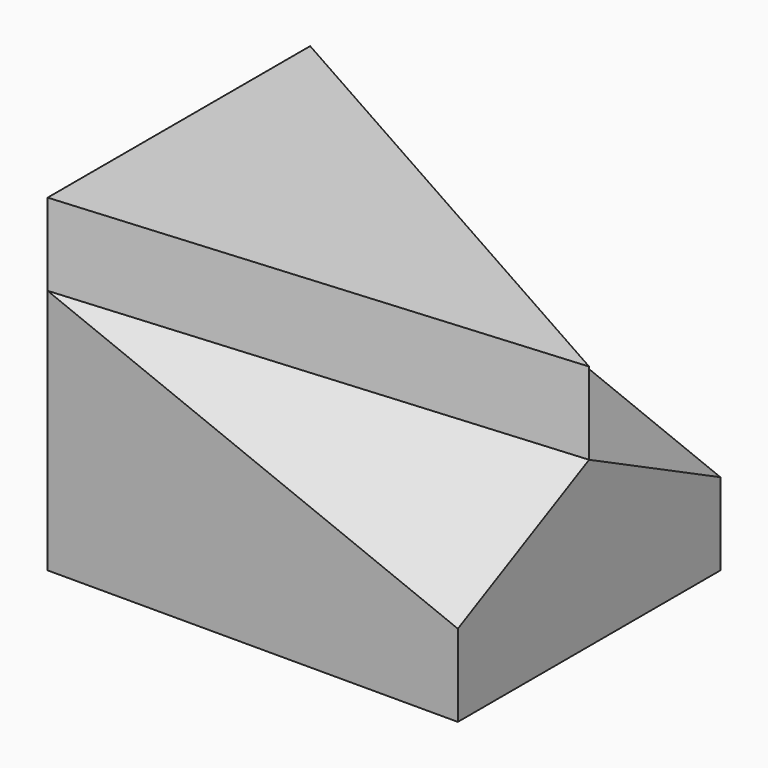
from build123d import *

# Parameters (mm, degrees)
F1_DEPTH = 20
F6_DEPTH = 16.8440384213


# Not quite as in the source:
# - a pattern or mirror of a feature is missing from the dataset's text; its kind, count and spacing are read off the source's solid
# - a feature names something its author has since deleted; it is built from what else it names


with BuildPart() as f1:
    # F0 (on Front) → F1 (new body, symmetric)
    with BuildSketch(Plane.XZ):
        Polygon((0, 30), (0, 0), (50, 0), (50, 20), align=None)
    extrude(amount=F1_DEPTH, both=True)

    # F5 (on 3pt) → F6 (cut, through all)
    with BuildSketch(Plane(origin=(11.3475177305, -14.1843971631, 28.3687943262), x_dir=(0.9415544714, 0.1506487154, -0.3012974309), z_dir=(-0.3368607684, 0.4210759605, -0.8421519211))):
        Polygon((41.0517749549, 13.416407865), (-12.0518972345, 4.472135955), (41.0517749549, -8.94427191), align=None)
    f6 = extrude(amount=-F6_DEPTH, mode=Mode.SUBTRACT)

    # F6_copies: F6 across plane
    add(f6.mirror(Plane.ZX), mode=Mode.SUBTRACT)

    # F8: sweep along a path in F7
    with BuildLine(Plane(origin=(0, 0, 0), x_dir=(0, -1, 0), z_dir=(-1, 0, 0))) as f8_path:
        Line((20, 30), (20, 40))
    # F1_face1 (on face) → F8 (sweep)
    with BuildSketch(Plane(origin=(16.6666666667, 0, 26.6666666667), x_dir=(1, 0, 0), z_dir=(0.1961161351, 0, 0.9805806757))):
        Polygon((-16.996731712, -20), (33.993463424, 0), (-16.996731712, 20), align=None)
    sweep(path=f8_path.line)


solid = f1.part
